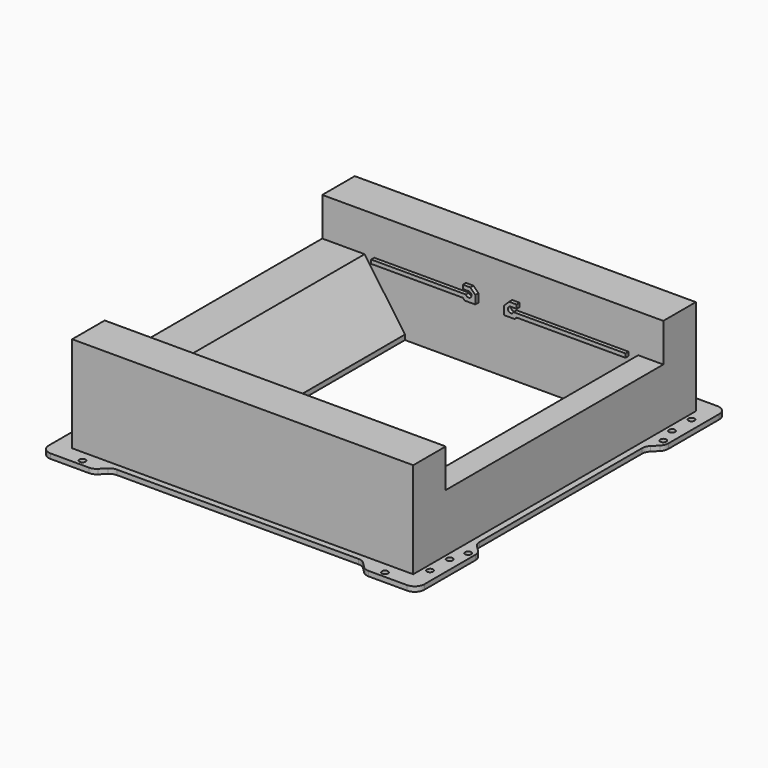
from build123d import *

# Parameters (mm, degrees)
F0_R     = 1.59
F0_W     = 91.44
F0_H     = 141.6
F1_DEPTH = 2.54
F3_DEPTH = 50
F5_DEPTH = 141.6
F7_DEPTH = 2


# Not quite as in the source:
# - a feature names something its author has since deleted; it is built from what else it names


with BuildPart() as f1:
    # F0 (on Top) → F1 (new body)
    with BuildSketch(Plane.XY):
        with BuildLine():
            ThreePointArc((0, 5), (1.4644660941, 1.4644660941), (5, 0))
            Line((5, 0), (25.0039321881, 0))
            ThreePointArc((25.0039321881, 0), (26.91734935, 0.3806023374), (28.5394660941, 1.4644660941))
            Line((28.5394660941, 1.4644660941), (31.3255339059, 4.2505339059))
            ThreePointArc((31.3255339059, 4.2505339059), (32.94765065, 5.3343976626), (34.8610678119, 5.715))
            Line((34.8610678119, 5.715), (160.7189321881, 5.715))
            ThreePointArc((160.7189321881, 5.715), (162.63234935, 5.3343976626), (164.2544660941, 4.2505339059))
            Line((164.2544660941, 4.2505339059), (167.0405339059, 1.4644660941))
            ThreePointArc((167.0405339059, 1.4644660941), (168.66265065, 0.3806023374), (170.5760678119, 0))
            Line((170.5760678119, 0), (190.58, 0))
            ThreePointArc((190.58, 0), (194.1155339059, 1.4644660941), (195.58, 5))
            Line((195.58, 5), (195.58, 38.1789321881))
            ThreePointArc((195.58, 38.1789321881), (195.1993976626, 40.09234935), (194.1155339059, 41.7144660941))
            Line((194.1155339059, 41.7144660941), (191.3294660941, 44.5005339059))
            ThreePointArc((191.3294660941, 44.5005339059), (190.2456023374, 46.12265065), (189.865, 48.0360678119))
            Line((189.865, 48.0360678119), (189.865, 153.8939321881))
            ThreePointArc((189.865, 153.8939321881), (190.2456023374, 155.80734935), (191.3294660941, 157.4294660941))
            Line((191.3294660941, 157.4294660941), (194.1155339059, 160.2155339059))
            ThreePointArc((194.1155339059, 160.2155339059), (195.1993976626, 161.83765065), (195.58, 163.7510678119))
            Line((195.58, 163.7510678119), (195.58, 196.93))
            ThreePointArc((195.58, 196.93), (194.1155339059, 200.4655339059), (190.58, 201.93))
            Line((190.58, 201.93), (170.5760678119, 201.93))
            ThreePointArc((170.5760678119, 201.93), (168.66265065, 201.5493976626), (167.0405339059, 200.4655339059))
            Line((167.0405339059, 200.4655339059), (164.2544660941, 197.6794660941))
            ThreePointArc((164.2544660941, 197.6794660941), (162.63234935, 196.5956023374), (160.7189321881, 196.215))
            Line((160.7189321881, 196.215), (34.8610678119, 196.215))
            ThreePointArc((34.8610678119, 196.215), (32.94765065, 196.5956023374), (31.3255339059, 197.6794660941))
            Line((31.3255339059, 197.6794660941), (28.5394660941, 200.4655339059))
            ThreePointArc((28.5394660941, 200.4655339059), (26.91734935, 201.5493976626), (25.0039321881, 201.93))
            Line((25.0039321881, 201.93), (5, 201.93))
            ThreePointArc((5, 201.93), (1.4644660941, 200.4655339059), (0, 196.93))
            Line((0, 196.93), (0, 163.7510678119))
            ThreePointArc((0, 163.7510678119), (0.3806023374, 161.83765065), (1.4644660941, 160.2155339059))
            Line((1.4644660941, 160.2155339059), (4.2505339059, 157.4294660941))
            ThreePointArc((4.2505339059, 157.4294660941), (5.3343976626, 155.80734935), (5.715, 153.8939321881))
            Line((5.715, 153.8939321881), (5.715, 48.0360678119))
            ThreePointArc((5.715, 48.0360678119), (5.3343976626, 46.12265065), (4.2505339059, 44.5005339059))
            Line((4.2505339059, 44.5005339059), (1.4644660941, 41.7144660941))
            ThreePointArc((1.4644660941, 41.7144660941), (0.3806023374, 40.09234935), (0, 38.1789321881))
            Line((0, 38.1789321881), (0, 5))
        make_face()
        with Locations((19.05, 3.175)):
            Circle(F0_R, mode=Mode.SUBTRACT)
        with Locations((5.715, 15.875)):
            Circle(F0_R, mode=Mode.SUBTRACT)
        with Locations((5.715, 28.575)):
            Circle(F0_R, mode=Mode.SUBTRACT)
        with Locations((3.175, 37.465)):
            Circle(F0_R, mode=Mode.SUBTRACT)
        with Locations((97.79, 100.965)):
            Rectangle(F0_W, F0_H, mode=Mode.SUBTRACT)
        with Locations((176.53, 3.175)):
            Circle(F0_R, mode=Mode.SUBTRACT)
        with Locations((189.865, 15.875)):
            Circle(F0_R, mode=Mode.SUBTRACT)
        with Locations((189.865, 28.575)):
            Circle(F0_R, mode=Mode.SUBTRACT)
        with Locations((192.405, 37.465)):
            Circle(F0_R, mode=Mode.SUBTRACT)
        with Locations((3.175, 164.465)):
            Circle(F0_R, mode=Mode.SUBTRACT)
        with Locations((5.715, 173.355)):
            Circle(F0_R, mode=Mode.SUBTRACT)
        with Locations((5.715, 186.055)):
            Circle(F0_R, mode=Mode.SUBTRACT)
        with Locations((19.05, 198.755)):
            Circle(F0_R, mode=Mode.SUBTRACT)
        with Locations((192.405, 164.465)):
            Circle(F0_R, mode=Mode.SUBTRACT)
        with Locations((189.865, 173.355)):
            Circle(F0_R, mode=Mode.SUBTRACT)
        with Locations((189.865, 186.055)):
            Circle(F0_R, mode=Mode.SUBTRACT)
        with Locations((176.53, 198.755)):
            Circle(F0_R, mode=Mode.SUBTRACT)
    extrude(amount=F1_DEPTH)

    # F2 (on face) → F3 (join)
    with BuildSketch(Plane.XY.offset(2.54)):
        Polygon((9, 192.93), (9, 171.765), (52.07, 171.765), (143.51, 171.765), (186.58, 171.765), (186.58, 192.93), align=None)
        Polygon((143.51, 30.165), (52.07, 30.165), (9, 30.165), (9, 9), (186.58, 9), (186.58, 30.165), align=None)
    extrude(amount=F3_DEPTH)

    # F4 (on face) → F5 (join, through all)
    with BuildSketch(Plane.XZ.offset(-171.765)):
        Polygon((9, 2.54), (52.07, 2.54), (31.0637738537, 32.54), (9, 32.54), align=None)
        Polygon((143.51, 2.54), (186.58, 2.54), (186.58, 32.54), (173.51, 32.54), align=None)
    extrude(amount=F5_DEPTH)

    # F6 (on face) → F7 (join)
    with BuildSketch(Plane.XZ.offset(-171.765)):
        with BuildLine():
            Line((105.29, 33.9308214303), (105.29, 29.54))
            Line((105.29, 29.54), (110.79, 29.54))
            Line((110.79, 29.54), (111.79, 30.54))
            Line((111.79, 30.54), (168.51, 30.54))
            Line((168.51, 30.54), (168.51, 32.54))
            Line((168.51, 32.54), (110.2042135624, 32.54))
            ThreePointArc((110.2042135624, 32.54), (107.5652551286, 32.1739745962), (108.79, 34.54))
            Line((108.79, 34.54), (111.79, 34.54))
            Line((111.79, 34.54), (111.79, 36.54))
            Line((111.79, 36.54), (107.8991785697, 36.54))
            Line((107.8991785697, 36.54), (105.29, 33.9308214303))
        make_face()
        with BuildLine():
            Line((36.0637738537, 30.54), (83.79, 30.54))
            Line((83.79, 30.54), (84.79, 29.54))
            Line((84.79, 29.54), (90.29, 29.54))
            Line((90.29, 29.54), (90.29, 33.9308214303))
            Line((90.29, 33.9308214303), (87.6808214303, 36.54))
            Line((87.6808214303, 36.54), (83.79, 36.54))
            Line((83.79, 36.54), (83.79, 34.54))
            Line((83.79, 34.54), (86.79, 34.54))
            ThreePointArc((86.79, 34.54), (88.0147448714, 32.1739745962), (85.3757864376, 32.54))
            Line((85.3757864376, 32.54), (36.0637738537, 32.54))
            Line((36.0637738537, 32.54), (36.0637738537, 30.54))
        make_face()
    extrude(amount=F7_DEPTH)


solid = f1.part
